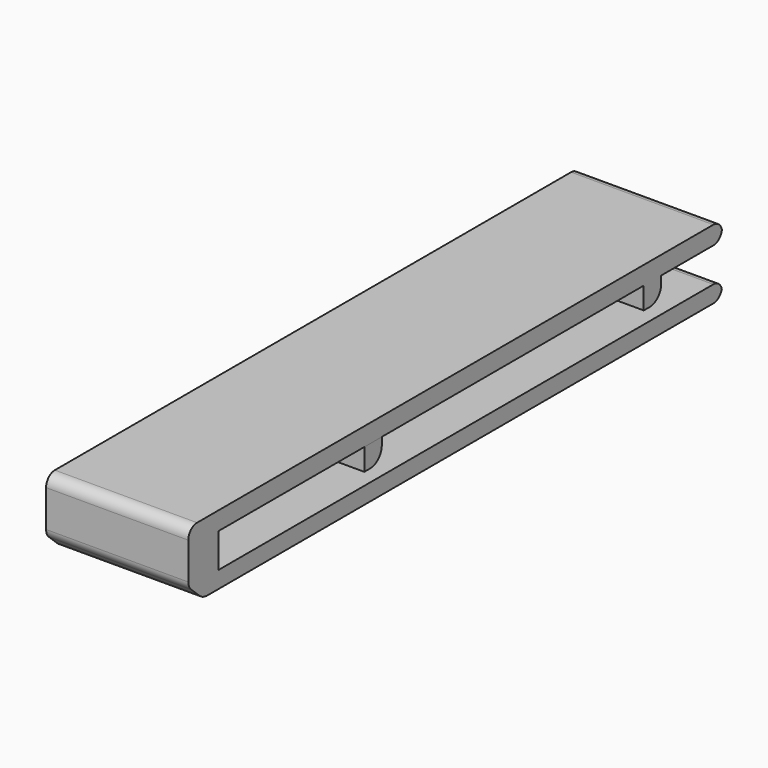
from build123d import *

# Parameters (mm, degrees)
F0_W        = 2.6942476507
F0_H        = 2.3
F0_W_2      = 86.3057523493
F0_H_2      = 2.5
F0_W_3      = 3
F0_H_3      = 3
F1_DEPTH    = 19.5
F2_T1_DEPTH = 27
F2_T3_DEPTH = 22.7585454732
F3_R        = 2
F3_2_R      = 2


# Not quite as in the source:
# - a fillet or chamfer that OpenCascade refuses, or shapes differently, is made with other operations: its cross-section is extruded or revolved along the edge and cut away or added


with BuildPart() as f1:
    # F0 (on Right) → F1 (new body)
    with BuildSketch(Plane.YZ):
        Polygon((-8.0138755839, 6.0200582189), (-8.0138755839, 1.3210557405), (-5.3196279332, 1.3210557405), (-5.3196279332, 6.0189673179), align=None)
        with Locations((-6.6667517586, 0.1710557405)):
            Rectangle(F0_W, F0_H)
        Polygon((-8.0138755839, -0.9789442595), (-8.0138755839, 1.3210557405), (-8.0138755839, 6.0200582189), (-10.4775000364, 6.0210557405), (-10.4775000364, 1.3210557405), align=None)
        with Locations((37.8332482414, 0.1710557405)):
            Rectangle(F0_W_2, F0_H)
        Polygon((-10.4775000364, 6.0210557405), (-8.0138755839, 6.0200582189), (-8.0138755839, 6.0210557405), align=None)
        Polygon((-8.0138755839, 6.0210557405), (-8.0138755839, 6.0200582189), (-5.3196279332, 6.0189673179), (-5.3196279332, 6.0210557405), align=None)
        Polygon((-5.3196279332, 6.0210557405), (-5.3196279332, 6.0189673179), (19.6803720668, 6.0088448171), (19.6803689531, 6.0210557405), (-2.3196279332, 6.0210557405), align=None)
        Polygon((-10.4775000364, 6.0210557405), (-8.0138755839, 6.0210557405), (-8.0138755839, 8.5210557405), (-10.4775000364, 8.5210557405), (-10.4775000364, 6.8358753532), align=None)
        with Locations((-6.6667517586, 7.2710557405)):
            Rectangle(F0_W, F0_H_2)
        with Locations((-3.8196279332, 7.2710557405)):
            Rectangle(F0_W_3, F0_H_2)
        Polygon((19.6803689531, 6.0210557405), (19.6803720668, 6.0088448171), (67.5681829453, 6.0210557405), align=None)
        Polygon((-2.3196279332, 8.5210557405), (-2.3196279332, 6.0210557405), (19.6803689531, 6.0210557405), (19.6797314776, 8.5210557405), align=None)
        Polygon((19.6803689531, 6.0210557405), (67.5681829453, 6.0210557405), (70.5681829453, 6.0210557405), (80.9861244161, 6.0210557405), (80.9861244161, 8.5210557405), (19.6797314776, 8.5210557405), align=None)
        with Locations((69.0681829453, 4.5210557405)):
            Rectangle(F0_W_3, F0_H_3)
    extrude(amount=F1_DEPTH)

    # F2: fillet of radius 1.5 on 6 edges, made by hand

    # F2_s2 → F2_t1 (cut)
    with BuildSketch(Plane.YZ.offset(-3.75)):
        with BuildLine():
            ThreePointArc((-8.9775000364, 8.5210557405), (-10.0381602081, 8.0817159123), (-10.4775000364, 7.0210557405))
            Line((-10.4775000364, 7.0210557405), (-10.4775000364, 8.5210557405))
            Line((-10.4775000364, 8.5210557405), (-8.9775000364, 8.5210557405))
        make_face()
        with BuildLine():
            ThreePointArc((80.9861244161, 7.0210557405), (80.5467845879, 8.0817159123), (79.4861244161, 8.5210557405))
            Line((79.4861244161, 8.5210557405), (80.9861244161, 8.5210557405))
            Line((80.9861244161, 8.5210557405), (80.9861244161, 7.0210557405))
        make_face()
        with BuildLine():
            ThreePointArc((79.4861244161, 6.0210557405), (80.5467845879, 6.4603955687), (80.9861244161, 7.5210557405))
            Line((80.9861244161, 7.5210557405), (80.9861244161, 6.0210557405))
            Line((80.9861244161, 6.0210557405), (79.4861244161, 6.0210557405))
        make_face()
        with BuildLine():
            ThreePointArc((80.9861244161, -0.1789442595), (80.5467845879, 0.8817159123), (79.4861244161, 1.3210557405))
            Line((79.4861244161, 1.3210557405), (80.9861244161, 1.3210557405))
            Line((80.9861244161, 1.3210557405), (80.9861244161, -0.1789442595))
        make_face()
        with BuildLine():
            ThreePointArc((79.4861244161, -0.9789442595), (80.5467845879, -0.5396044313), (80.9861244161, 0.5210557405))
            Line((80.9861244161, 0.5210557405), (80.9861244161, -0.9789442595))
            Line((80.9861244161, -0.9789442595), (79.4861244161, -0.9789442595))
        make_face()
    extrude(amount=F2_T1_DEPTH, mode=Mode.SUBTRACT)

    # F2_s4 → F2_t3 (cut)
    with BuildSketch(Plane.YZ.offset(-1.6292727366)):
        with BuildLine():
            ThreePointArc((-10.0011242018, 0.8763189551), (-10.3532609618, 1.3750342303), (-10.4775000364, 1.9727648351))
            Line((-10.4775000364, 1.9727648351), (-10.4775000364, 1.3210557405))
            Line((-10.4775000364, 1.3210557405), (-10.0011242018, 0.8763189551))
        make_face()
    extrude(amount=F2_T3_DEPTH, mode=Mode.SUBTRACT)

    # F3
    f3_edges = [f1.edges().sort_by_distance(p)[0] for p in [
        (9.75, -8.013876, -0.978944),
        (9.75, 70.568183, 3.021056),
    ]]
    fillet(f3_edges, radius=F3_R)


with BuildPart() as f1b:
    # F0 (on Right) → F1, piece 2 (new body)
    with BuildSketch(Plane.YZ):
        with Locations((21.1803720668, 4.5088448171)):
            Rectangle(F0_W_3, F0_H_3)
    extrude(amount=F1_DEPTH)

    # F3#2
    f3_2_edges = [f1b.edges().sort_by_distance(p)[0] for p in [
        (9.75, 22.680372, 3.008845),
    ]]
    fillet(f3_2_edges, radius=F3_2_R)


solid = Compound([f1.part, f1b.part])
